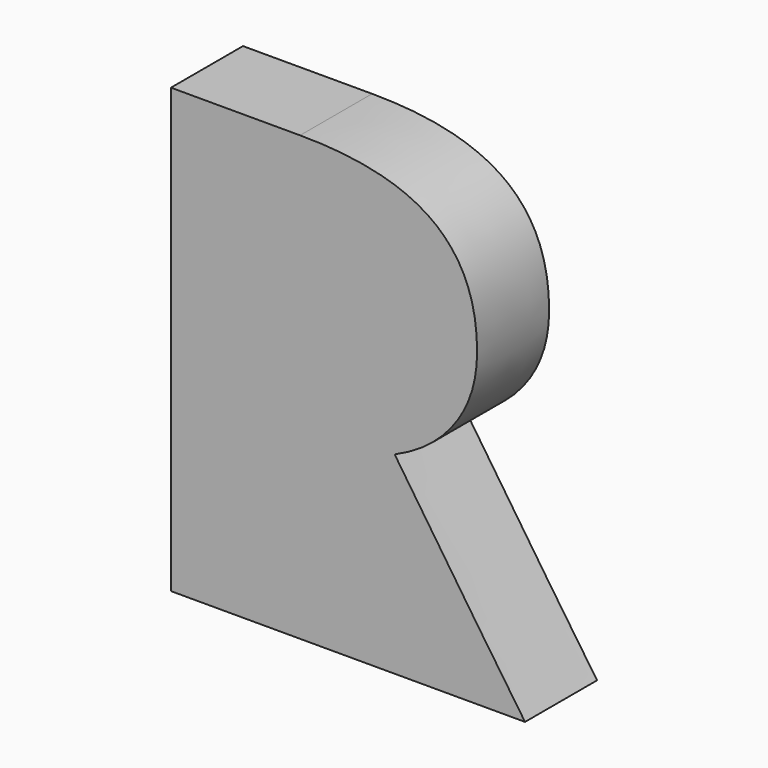
from build123d import *

# Parameters (mm, degrees)
F0_TEXT_SIZE = 6.8965517241
F1_DEPTH     = 1


# Not quite as in the source:
# - Text() gives the source's letters only with a copy of the font that has no kerning and outlines rounded to 1/6400 em; it was checked with that copy


with BuildPart() as f1:
    # F0 (on Front) → F1 (new body)
    with BuildSketch(Plane.XZ):
        with Locations((-2.5, -2.7556776304)):
            Text('R', F0_TEXT_SIZE, font='Open Sans', font_style=FontStyle.BOLD, text_align=(TextAlign.LEFT, TextAlign.BOTTOM))
        with BuildLine():
            Line((-0.8362068966, 1.3122103007), (-0.8362068966, -0.0175310787))
            Line((-0.8362068966, -0.0175310787), (-0.5, -0.0175310787))
            add(Edge.make_bspline(
                [(-0.5, -0.0175310787), (-0.0043103448, -0.0175310787), (0.2311422414, 0.147339611)],
                knots=[0, 0, 0, 1, 1, 1], degree=2))
            add(Edge.make_bspline(
                [(0.2311422414, 0.147339611), (0.4665948276, 0.3122103007), (0.4665948276, 0.6656585765)],
                knots=[0, 0, 0, 1, 1, 1], degree=2))
            add(Edge.make_bspline(
                [(0.4665948276, 0.6656585765), (0.4665948276, 1.0158740938), (0.2257543103, 1.1640421972)],
                knots=[0, 0, 0, 1, 1, 1], degree=2))
            add(Edge.make_bspline(
                [(0.2257543103, 1.1640421972), (-0.0150862069, 1.3122103007), (-0.5193965517, 1.3122103007)],
                knots=[0, 0, 0, 1, 1, 1], degree=2))
            Line((-0.5193965517, 1.3122103007), (-0.8362068966, 1.3122103007))
        make_face()
        Polygon((-0.8362068966, -0.8666690097), (-0.8362068966, -2.7556776304), (0.8943965517, -2.7556776304), (-0.28125, -0.8666690097), align=None)
    extrude(amount=-F1_DEPTH)


solid = f1.part
